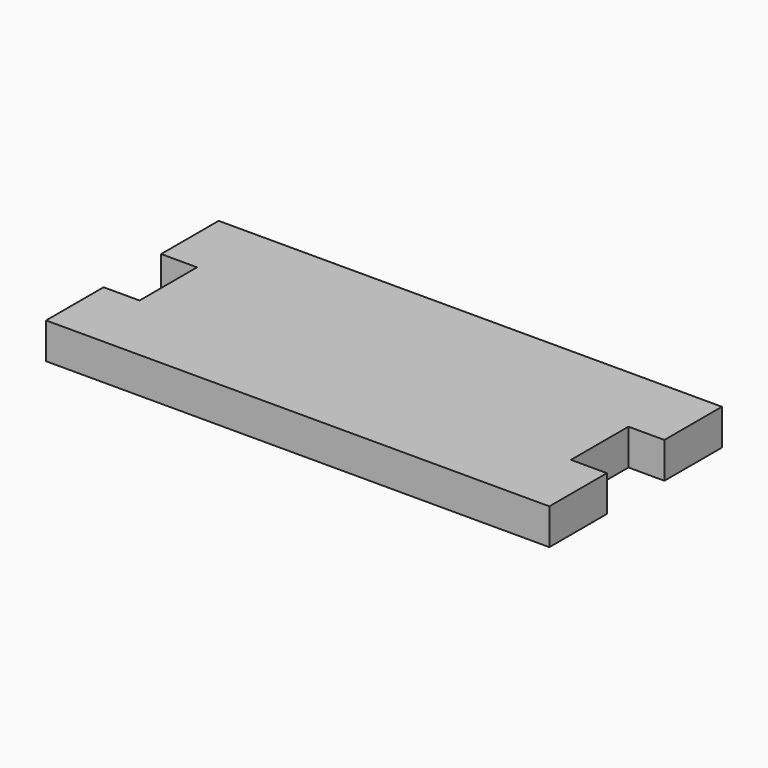
from build123d import *

# Parameters (mm, degrees)
F1_DEPTH = 6.35


# Not quite as in the source:
# - a feature names something its author has since deleted; it is built from what else it names


with BuildPart() as f1:
    # F0 (on Top) → F1 (new body)
    with BuildSketch(Plane.XY):
        Polygon((44.45, 19.05), (38.1, 19.05), (-38.1, 19.05), (-44.45, 19.05), (-44.45, 6.35), (-38.1, 6.35), (-38.1, -6.35), (-44.45, -6.35), (-44.45, -19.05), (-38.1, -19.05), (38.1, -19.05), (44.45, -19.05), (44.45, -6.35), (38.1, -6.35), (38.1, 6.35), (44.45, 6.35), align=None)
    extrude(amount=F1_DEPTH)


solid = f1.part
